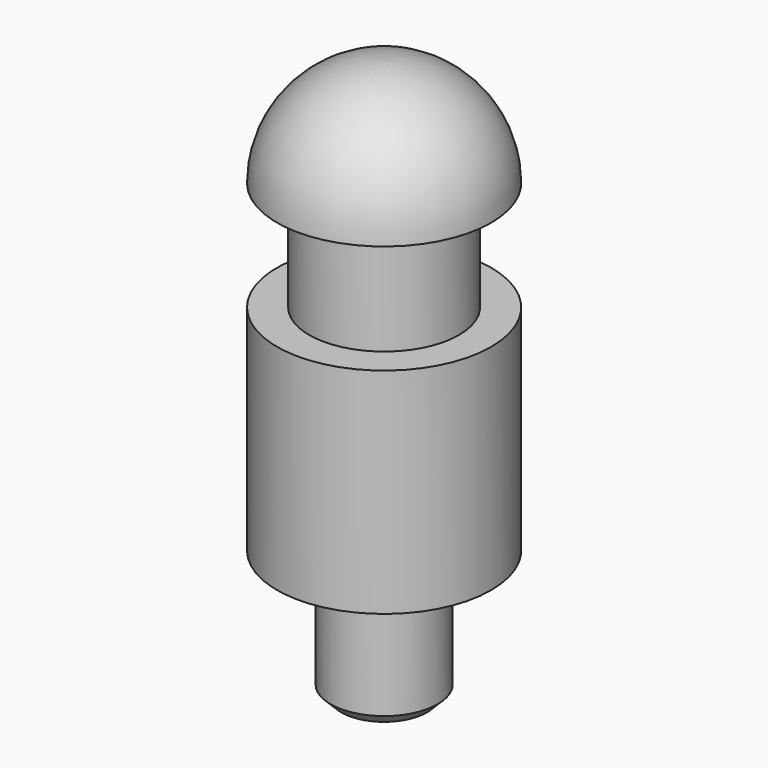
from build123d import *

# Parameters (mm, degrees)
F0_R     = 2.5
F1_DEPTH = 6
F2_R     = 5
F3_DEPTH = 10
F4_R     = 3.5
F5_DEPTH = 5.1
F6_R     = 5
F7_DEPTH = 5
F8_SIZE  = 0.5
F9_R     = 4.99999


# Not quite as in the source:
# - a fillet or chamfer is up to 0.001 mm smaller than in the source, because OpenCascade refuses the exact size


with BuildPart() as f1:
    # F0 (on Top) → F1 (new body)
    with BuildSketch(Plane.XY):
        Circle(F0_R)
    extrude(amount=F1_DEPTH)

    # F2 (on face) → F3 (join)
    with BuildSketch(Plane.XY.offset(6)):
        Circle(F2_R)
    extrude(amount=F3_DEPTH)

    # F4 (on face) → F5 (join)
    with BuildSketch(Plane.XY.offset(16)):
        Circle(F4_R)
    extrude(amount=F5_DEPTH)

    # F6 (on face) → F7 (join)
    with BuildSketch(Plane.XY.offset(21.1)):
        Circle(F6_R)
    extrude(amount=F7_DEPTH)

    # F8
    f8_edges = [f1.edges().sort_by_distance(p)[0] for p in [
        (-2.5, 0, 0),
    ]]
    chamfer(f8_edges, length=F8_SIZE)

    # F9 (radius 5 in the source; OpenCascade refuses exactly that, so slightly less here)
    f9_edges = [f1.edges().sort_by_distance(p)[0] for p in [
        (-5, 0, 26.1),
    ]]
    fillet(f9_edges, radius=F9_R)


solid = f1.part
